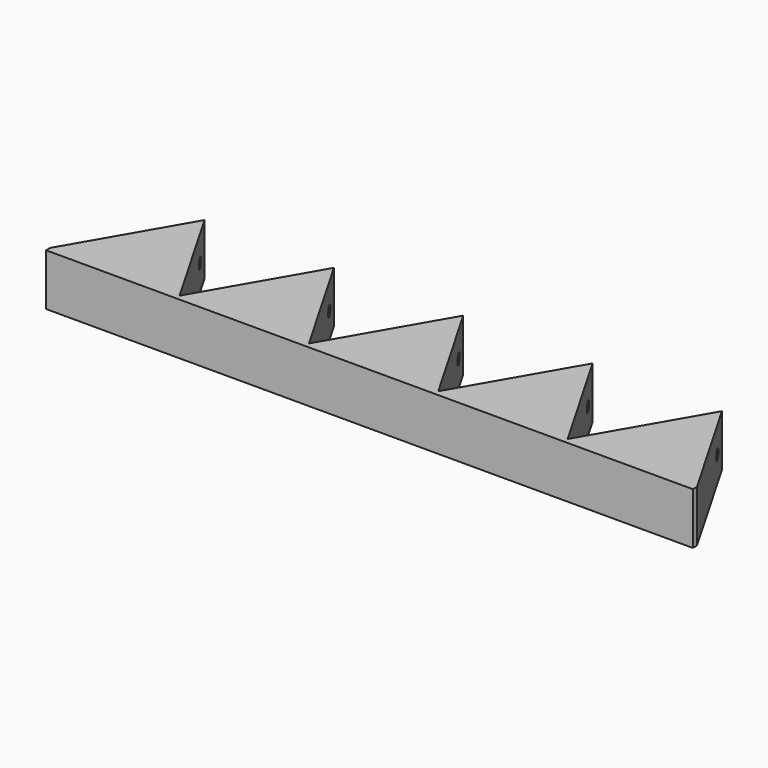
from build123d import *

# Parameters (mm, degrees)
F1_DEPTH    = 10
F2_T        = 2
F2_T3_DEPTH = 14
F3_R        = 1
F4_DEPTH    = 100


# Not quite as in the source:
# - a shell that OpenCascade refuses in one call is made with other operations: the cavity is built on its own and cut out


with BuildPart() as f1:
    # F0 (on Top) → F1 (new body)
    with BuildSketch(Plane.XY):
        Polygon((-50, 0), (-25, 0), (-37.5, 21.6506350946), align=None)
        Polygon((-12.5, 21.6506350946), (-25, 0), (0, 0), align=None)
        Polygon((12.5, 21.6506350946), (0, 0), (25, 0), align=None)
        Polygon((37.5, 21.6506350946), (25, 0), (50, 0), align=None)
        Polygon((62.5, 21.6506350946), (50, 0), (75, 0), align=None)
        Polygon((0, 0), (-25, 0), (-50, 0), (-50, -1), (75, -1), (75, 0), (50, 0), (25, 0), align=None)
    extrude(amount=F1_DEPTH)

    # F2: shell of thickness 2, made by hand


with BuildPart() as f2_core1:
    # F2_t2: copy of F1
    add(f1.part)

    # the walls: a layer under each face that stays
    f2_faces = [f2_core1.faces().sort_by_distance(p)[0] for p in [
        (-31.25, 10.8253175473, 5),
        (-43.75, 10.8253175473, 5),
        (-50, -0.5, 5),
        (12.5, -1, 5),
        (75, -0.5, 5),
        (68.75, 10.8253175473, 5),
        (56.25, 10.8253175473, 5),
        (43.75, 10.8253175473, 5),
        (31.25, 10.8253175473, 5),
        (18.75, 10.8253175473, 5),
        (6.25, 10.8253175473, 5),
        (-6.25, 10.8253175473, 5),
        (-18.75, 10.8253175473, 5),
        (12.5, 10.3253175473, 0),
        (12.5, 10.3253175473, 10),
    ]]
    thicken(f2_faces, amount=-F2_T, mode=Mode.SUBTRACT)

    # F2_s4 → F2_t3 (cut)
    with BuildSketch(Plane.XY.offset(-2)):
        Polygon((-25, 0.02), (-26.7320508076, -1), (-25, -4), (-23.2679491924, -1), align=None)
        Polygon((50, 0.02), (51.7320508076, -1), (50, -4), (48.2679491924, -1), align=None)
        Polygon((25, 0.02), (26.7320508076, -1), (25, -4), (23.2679491924, -1), align=None)
        Polygon((0, 0.02), (1.7320508076, -1), (0, -4), (-1.7320508076, -1), align=None)
    extrude(amount=F2_T3_DEPTH, mode=Mode.SUBTRACT)


with BuildPart() as f1_1:
    add(f1.part)

    # what is left inside the walls is the cavity
    f2_cavity = [f2_core1.part.solids().sort_by_distance(p)[0] for p in [
        (-37.5, 6.550212, 2.02),
        (-12.5, 6.550212, 2.02),
        (12.5, 6.550212, 2.02),
        (37.5, 6.550212, 2.02),
        (62.5, 6.550212, 2.02),
    ]]
    add(f2_cavity, mode=Mode.SUBTRACT)

    # F3 (on Right) → F4 (cut, symmetric)
    with BuildSketch(Plane.YZ):
        with Locations((17.6506350946, 5)):
            Circle(F3_R)
    extrude(amount=F4_DEPTH, both=True, mode=Mode.SUBTRACT)


solid = f1_1.part
